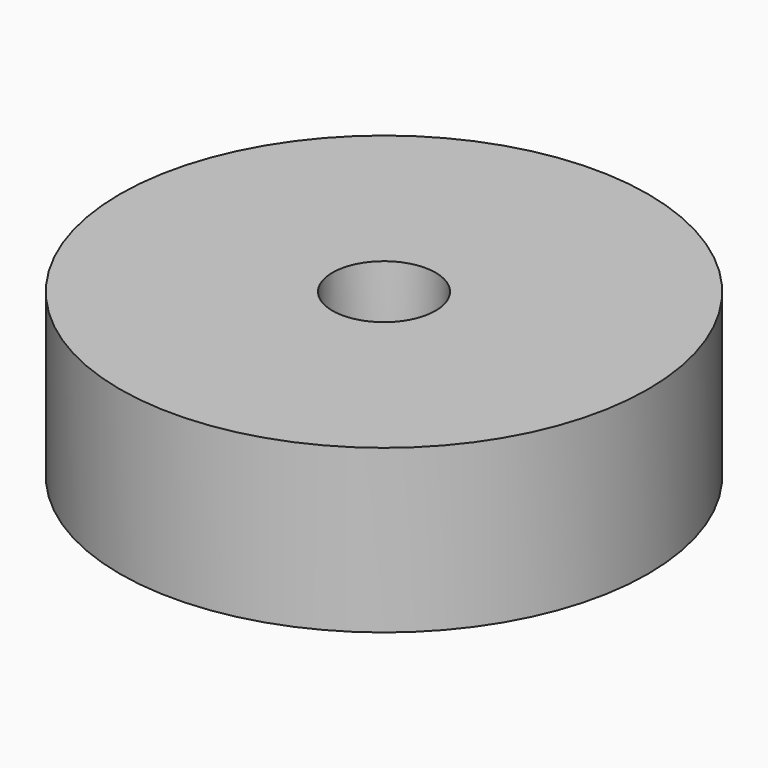
from build123d import *

# Parameters (mm, degrees)
F0_R     = 32.5
F0_R_2   = 5.85
F1_DEPTH = 20
F2_SIZE2 = 0.49999
F2_SIZE  = 19.99999


# Not quite as in the source:
# - a fillet or chamfer is up to 0.001 mm smaller than in the source, because OpenCascade refuses the exact size


with BuildPart() as f1:
    # F0 (on Top) → F1 (new body)
    with BuildSketch(Plane.XY):
        Circle(F0_R)
        Circle(F0_R_2, mode=Mode.SUBTRACT)
    extrude(amount=F1_DEPTH)

    # F2 (size 20 and 0.5 in the source; OpenCascade refuses exactly that, so slightly less here)
    f2_edges = [f1.edges().sort_by_distance(p)[0] for p in [
        (-5.85, 0, 20),
    ]]
    f2_side = f1.faces().sort_by_distance((-5.85, 0, 10))[0]
    chamfer(f2_edges, length=F2_SIZE, length2=F2_SIZE2, reference=f2_side)


solid = f1.part
